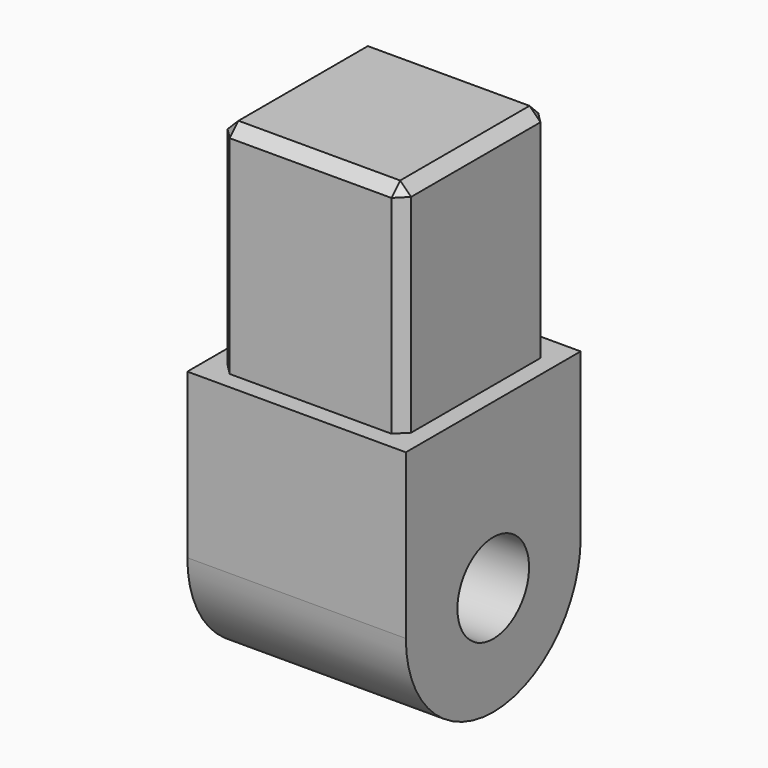
from build123d import *

# Parameters (mm, degrees)
F0_W     = 20
F0_H     = 20
F1_DEPTH = 25
F2_W     = 16.8
F2_H     = 16.8
F3_DEPTH = 20
F4_SIZE  = 1
F5_R     = 9.99999
F7_D     = 8.2
F7_DEPTH = 35
F7_TIP   = 2.463528538


# Not quite as in the source:
# - a fillet or chamfer is up to 0.001 mm smaller than in the source, because OpenCascade refuses the exact size


with BuildPart() as f1:
    # F0 (on Top) → F1 (new body)
    with BuildSketch(Plane.XY):
        with Locations((15, 10)):
            Rectangle(F0_W, F0_H)
    extrude(amount=F1_DEPTH)

    # F2 (on face) → F3 (join)
    with BuildSketch(Plane.XY.offset(25)):
        with Locations((15, 10)):
            Rectangle(F2_W, F2_H)
    extrude(amount=F3_DEPTH)

    # F4
    f4_edges = [f1.edges().sort_by_distance(p)[0] for p in [
        (6.6, 18.4, 35),
        (6.6, 10, 45),
        (15, 18.4, 45),
        (23.4, 18.4, 35),
        (23.4, 10, 45),
        (15, 1.6, 45),
        (6.6, 1.6, 35),
        (23.4, 1.6, 35),
    ]]
    chamfer(f4_edges, length=F4_SIZE)

    # F5 (radius 10 in the source; OpenCascade refuses exactly that, so slightly less here)
    f5_edges = [f1.edges().sort_by_distance(p)[0] for p in [
        (15, 0, 0),
        (15, 20, 0),
    ]]
    fillet(f5_edges, radius=F5_R)

    # F7
    with Locations(Plane.YZ.offset(25)):
        with Locations((10, 10)):
            Hole(F7_D / 2, depth=F7_DEPTH)
            with Locations((0, 0, -(F7_DEPTH + F7_TIP / 2))):  # 118° drill point
                Cone(0, F7_D / 2, F7_TIP, mode=Mode.SUBTRACT)


solid = f1.part
